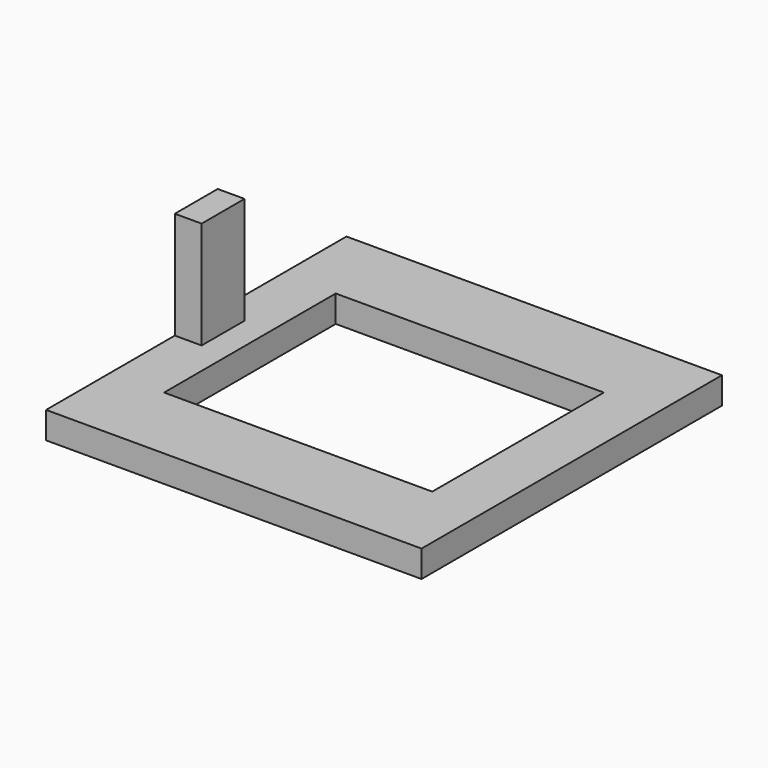
from build123d import *

# Parameters (mm, degrees)
F0_W     = 70
F0_H     = 70
F0_W_2   = 50
F0_H_2   = 40
F1_DEPTH = 5
F2_W     = 5
F2_H     = 10
F3_DEPTH = 25


# Not quite as in the source:
# - a feature names something its author has since deleted; it is built from what else it names


with BuildPart() as f1:
    # F0 (on Top) → F1 (new body)
    with BuildSketch(Plane.XY):
        with Locations((35, 35)):
            Rectangle(F0_W, F0_H)
        with Locations((35, 35)):
            Rectangle(F0_W_2, F0_H_2, mode=Mode.SUBTRACT)
    extrude(amount=F1_DEPTH)

    # F2 (on Top) → F3 (join)
    with BuildSketch(Plane.XY):
        with Locations((2.5, 35)):
            Rectangle(F2_W, F2_H)
    extrude(amount=F3_DEPTH)


solid = f1.part
